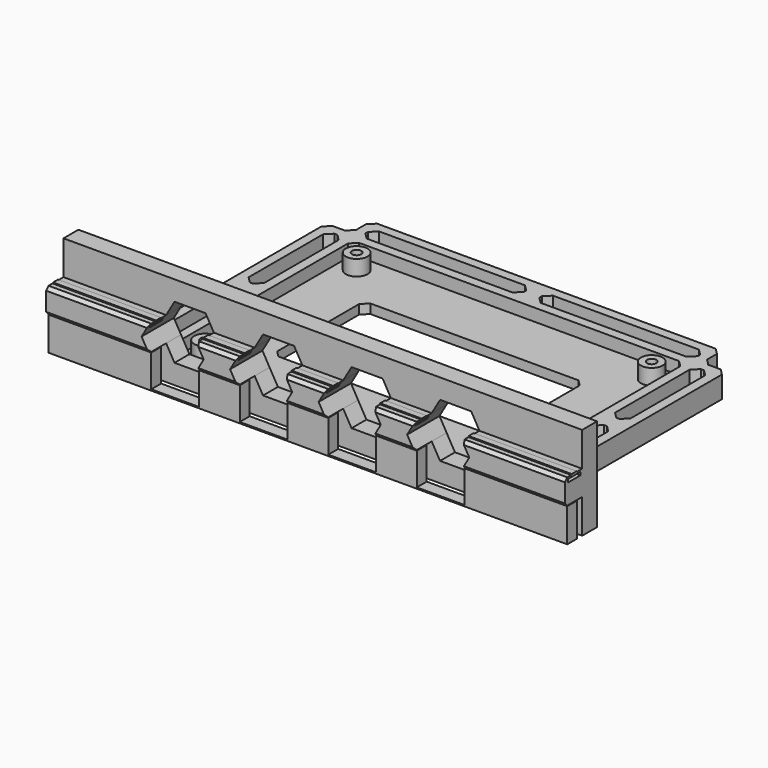
from build123d import *

# Parameters (mm, degrees)
F0_W      = 107
F0_H      = 73
F0_R      = 3.5
F0_W_2    = 71
F0_H_2    = 37
F0_R_2    = 1.5
F0_W_3    = 5
F0_H_3    = 5
F0_W_4    = 3
F0_H_4    = 3
F1_DEPTH  = 3
F2_DEPTH  = 4
F3_DEPTH  = 5
F4_DEPTH  = 27
F6_DEPTH  = 6
F5_W      = 7.5
F5_H      = 8
F5_R      = 3.05
F7_DEPTH  = 7
F8_SIZE   = 1
F9_SIZE   = 2
F11_DEPTH = 167
F12_DEPTH = 7.001
F10_W     = 5
F10_H     = 1
F13_DEPTH = 167.001
F14_W     = 33.0594010768
F14_H     = 4
F14_W_2   = 15.3811978465
F14_W_3   = 13.1188021535
F15_DEPTH = 0.4
F16_DEPTH = 10.8


# Not quite as in the source:
# - an extrude ends at something that could not be found from the text; its depth is read off the source's solid


with BuildPart() as f1:
    # F0 (on Top) → F1 (new body)
    with BuildSketch(Plane.XY):
        Rectangle(F0_W, F0_H)
        with Locations((-47.5, -30.5)):
            Circle(F0_R, mode=Mode.SUBTRACT)
        with Locations((47.5, -30.5)):
            Circle(F0_R, mode=Mode.SUBTRACT)
        Rectangle(F0_W_2, F0_H_2, mode=Mode.SUBTRACT)
        with Locations((-47.5, 30.5)):
            Circle(F0_R, mode=Mode.SUBTRACT)
        with Locations((47.5, 30.5)):
            Circle(F0_R, mode=Mode.SUBTRACT)
        with Locations((-47.5, 30.5)):
            Circle(F0_R)
        with Locations((-47.5, 30.5)):
            Circle(F0_R_2, mode=Mode.SUBTRACT)
        with Locations((-47.5, -30.5)):
            Circle(F0_R)
        with Locations((-47.5, -30.5)):
            Circle(F0_R_2, mode=Mode.SUBTRACT)
        with Locations((47.5, -30.5)):
            Circle(F0_R)
        with Locations((47.5, -30.5)):
            Circle(F0_R_2, mode=Mode.SUBTRACT)
        with Locations((47.5, 30.5)):
            Circle(F0_R)
        with Locations((47.5, 30.5)):
            Circle(F0_R_2, mode=Mode.SUBTRACT)
        Polygon((-53.5, -36.5), (-53.5, 36.5), (-56.5, 36.5), (-56.5, 2.5), (-56.5, -2.5), (-56.5, -36.5), align=None)
        Polygon((-56.5, 36.5), (-56.5, 39.5), (-64.5, 39.5), (-64.5, -36.5), (-61.5, -36.5), (-61.5, -2.5), (-61.5, 2.5), (-61.5, 36.5), align=None)
        with Locations((-59, 0)):
            Rectangle(F0_W_3, F0_H_3)
        with Locations((-55, 38)):
            Rectangle(F0_W_4, F0_H_4)
        Polygon((-53.5, 39.5), (-53.5, 44.5), (-2.5, 44.5), (2.5, 44.5), (53.5, 44.5), (53.5, 39.5), (56.5, 39.5), (56.5, 47.5), (-56.5, 47.5), (-56.5, 39.5), align=None)
        Polygon((-2.5, 39.5), (-53.5, 39.5), (-53.5, 36.5), (53.5, 36.5), (53.5, 39.5), (2.5, 39.5), align=None)
        Polygon((53.5, -36.5), (-53.5, -36.5), (-56.5, -36.5), (-61.5, -36.5), (-64.5, -36.5), (-83.5, -36.5), (-83.5, -42.5), (83.5, -42.5), (83.5, -36.5), (64.5, -36.5), (61.5, -36.5), (56.5, -36.5), align=None)
        with Locations((0, 42)):
            Rectangle(F0_W_3, F0_H_3)
        with Locations((55, 38)):
            Rectangle(F0_W_4, F0_H_4)
        Polygon((56.5, 39.5), (56.5, 36.5), (61.5, 36.5), (61.5, 2.5), (61.5, -2.5), (61.5, -36.5), (64.5, -36.5), (64.5, 39.5), align=None)
        with Locations((59, 0)):
            Rectangle(F0_W_3, F0_H_3)
        Polygon((56.5, 36.5), (53.5, 36.5), (53.5, -36.5), (56.5, -36.5), (56.5, -2.5), (56.5, 2.5), align=None)
    extrude(amount=-F1_DEPTH)

    # F0 (on Top) → F2 (join)
    with BuildSketch(Plane.XY):
        Polygon((-53.5, -36.5), (-53.5, 36.5), (-56.5, 36.5), (-56.5, 2.5), (-56.5, -2.5), (-56.5, -36.5), align=None)
        with Locations((-55, 38)):
            Rectangle(F0_W_4, F0_H_4)
        Polygon((-53.5, 39.5), (-53.5, 44.5), (-2.5, 44.5), (2.5, 44.5), (53.5, 44.5), (53.5, 39.5), (56.5, 39.5), (56.5, 47.5), (-56.5, 47.5), (-56.5, 39.5), align=None)
        Polygon((-56.5, 36.5), (-56.5, 39.5), (-64.5, 39.5), (-64.5, -36.5), (-61.5, -36.5), (-61.5, -2.5), (-61.5, 2.5), (-61.5, 36.5), align=None)
        with Locations((-59, 0)):
            Rectangle(F0_W_3, F0_H_3)
        with Locations((0, 42)):
            Rectangle(F0_W_3, F0_H_3)
        Polygon((-2.5, 39.5), (-53.5, 39.5), (-53.5, 36.5), (53.5, 36.5), (53.5, 39.5), (2.5, 39.5), align=None)
        with Locations((55, 38)):
            Rectangle(F0_W_4, F0_H_4)
        Polygon((56.5, 36.5), (53.5, 36.5), (53.5, -36.5), (56.5, -36.5), (56.5, -2.5), (56.5, 2.5), align=None)
        Polygon((56.5, 39.5), (56.5, 36.5), (61.5, 36.5), (61.5, 2.5), (61.5, -2.5), (61.5, -36.5), (64.5, -36.5), (64.5, 39.5), align=None)
        with Locations((59, 0)):
            Rectangle(F0_W_3, F0_H_3)
    extrude(amount=F2_DEPTH)

    # F0 (on Top) → F3 (join)
    with BuildSketch(Plane.XY):
        with Locations((-47.5, 30.5)):
            Circle(F0_R)
        with Locations((-47.5, 30.5)):
            Circle(F0_R_2, mode=Mode.SUBTRACT)
        with Locations((47.5, 30.5)):
            Circle(F0_R)
        with Locations((47.5, 30.5)):
            Circle(F0_R_2, mode=Mode.SUBTRACT)
        with Locations((47.5, -30.5)):
            Circle(F0_R)
        with Locations((47.5, -30.5)):
            Circle(F0_R_2, mode=Mode.SUBTRACT)
        with Locations((-47.5, -30.5)):
            Circle(F0_R)
        with Locations((-47.5, -30.5)):
            Circle(F0_R_2, mode=Mode.SUBTRACT)
    extrude(amount=F3_DEPTH)

    # F0 (on Top) → F4 (join)
    with BuildSketch(Plane.XY):
        Polygon((53.5, -36.5), (-53.5, -36.5), (-56.5, -36.5), (-61.5, -36.5), (-64.5, -36.5), (-83.5, -36.5), (-83.5, -42.5), (83.5, -42.5), (83.5, -36.5), (64.5, -36.5), (61.5, -36.5), (56.5, -36.5), align=None)
    extrude(amount=F4_DEPTH)

    # F5 (on face) → F6 (cut, through all)
    with BuildSketch(Plane.XZ.offset(42.5)):
        Polygon((-47.75, 20.6602540378), (-50.4405989232, 16), (-35.0594010768, 16), (-37.75, 20.6602540378), align=None)
        Polygon((-35.0594010768, 16), (-50.4405989232, 16), (-52.75, 12), (-50.4405989232, 8), (-35.0594010768, 8), (-32.75, 12), align=None)
        Polygon((-35.0594010768, 8), (-50.4405989232, 8), (-47.75, 3.3397459622), (-37.75, 3.3397459622), align=None)
        Polygon((-6.5594010768, 8), (-21.9405989232, 8), (-19.25, 3.3397459622), (-9.25, 3.3397459622), align=None)
        Polygon((-6.5594010768, 16), (-21.9405989232, 16), (-24.25, 12), (-21.9405989232, 8), (-6.5594010768, 8), (-4.25, 12), align=None)
        Polygon((-19.25, 20.6602540378), (-21.9405989232, 16), (-6.5594010768, 16), (-9.25, 20.6602540378), align=None)
        Polygon((9.25, 20.6602540378), (6.5594010768, 16), (21.9405989232, 16), (19.25, 20.6602540378), align=None)
        Polygon((21.9405989232, 16), (6.5594010768, 16), (4.25, 12), (6.5594010768, 8), (21.9405989232, 8), (24.25, 12), align=None)
        Polygon((21.9405989232, 8), (6.5594010768, 8), (9.25, 3.3397459622), (19.25, 3.3397459622), align=None)
        Polygon((47.75, 3.3397459622), (50.4405989232, 8), (35.0594010768, 8), (37.75, 3.3397459622), align=None)
        Polygon((52.75, 12), (50.4405989232, 16), (35.0594010768, 16), (32.75, 12), (35.0594010768, 8), (50.4405989232, 8), align=None)
        Polygon((35.0594010768, 16), (50.4405989232, 16), (47.75, 20.6602540378), (37.75, 20.6602540378), align=None)
    extrude(amount=-F6_DEPTH, mode=Mode.SUBTRACT)

    # F5 (on face) → F7 (join)
    with BuildSketch(Plane.XZ.offset(42.5)):
        with Locations((-79.75, 12)):
            Rectangle(F5_W, F5_H)
        with Locations((79.75, 12)):
            Rectangle(F5_W, F5_H)
        Polygon((61, 8), (61, 16), (50.4405989232, 16), (52.75, 12), (50.4405989232, 8), align=None)
        Polygon((32.75, 12), (35.0594010768, 16), (21.9405989232, 16), (24.25, 12), (21.9405989232, 8), (35.0594010768, 8), align=None)
        Polygon((6.5594010768, 16), (-6.5594010768, 16), (-4.25, 12), (-6.5594010768, 8), (6.5594010768, 8), (4.25, 12), align=None)
        Polygon((-21.9405989232, 16), (-35.0594010768, 16), (-32.75, 12), (-35.0594010768, 8), (-21.9405989232, 8), (-24.25, 12), align=None)
        Polygon((-50.4405989232, 16), (-61, 16), (-61, 8), (-50.4405989232, 8), (-52.75, 12), align=None)
        with BuildLine():
            ThreePointArc((64.5808164115, 8), (62.9, 12), (64.5808164115, 16))
            Line((64.5808164115, 16), (61, 16))
            Line((61, 16), (61, 8))
            Line((61, 8), (64.5808164115, 8))
        make_face()
        with BuildLine():
            ThreePointArc((74.1, 12), (73.6627235107, 14.1693976013), (72.4191835885, 16))
            Line((72.4191835885, 16), (64.5808164115, 16))
            ThreePointArc((64.5808164115, 16), (62.9, 12), (64.5808164115, 8))
            Line((64.5808164115, 8), (72.4191835885, 8))
            ThreePointArc((72.4191835885, 8), (73.6627235107, 9.8306023987), (74.1, 12))
        make_face()
        with Locations((68.5, 12)):
            Circle(F5_R, mode=Mode.SUBTRACT)
        with Locations((68.5, 12)):
            Circle(F5_R)
        with BuildLine():
            Line((76, 8), (76, 16))
            Line((76, 16), (72.4191835885, 16))
            ThreePointArc((72.4191835885, 16), (73.6627235107, 14.1693976013), (74.1, 12))
            ThreePointArc((74.1, 12), (73.6627235107, 9.8306023987), (72.4191835885, 8))
            Line((72.4191835885, 8), (76, 8))
        make_face()
        with BuildLine():
            Line((-61, 16), (-64.5808164115, 16))
            ThreePointArc((-64.5808164115, 16), (-63.3372764893, 14.1693976013), (-62.9, 12))
            ThreePointArc((-62.9, 12), (-63.3372764893, 9.8306023987), (-64.5808164115, 8))
            Line((-64.5808164115, 8), (-61, 8))
            Line((-61, 8), (-61, 16))
        make_face()
        with BuildLine():
            Line((-64.5808164115, 16), (-72.4191835885, 16))
            ThreePointArc((-72.4191835885, 16), (-74.1, 12), (-72.4191835885, 8))
            Line((-72.4191835885, 8), (-64.5808164115, 8))
            ThreePointArc((-64.5808164115, 8), (-63.3372764893, 9.8306023987), (-62.9, 12))
            ThreePointArc((-62.9, 12), (-63.3372764893, 14.1693976013), (-64.5808164115, 16))
        make_face()
        with Locations((-68.5, 12)):
            Circle(F5_R, mode=Mode.SUBTRACT)
        with Locations((-68.5, 12)):
            Circle(F5_R)
        with BuildLine():
            Line((-72.4191835885, 16), (-76, 16))
            Line((-76, 16), (-76, 8))
            Line((-76, 8), (-72.4191835885, 8))
            ThreePointArc((-72.4191835885, 8), (-74.1, 12), (-72.4191835885, 16))
        make_face()
    extrude(amount=F7_DEPTH)

    # F8
    f8_edges = [f1.edges().sort_by_distance(p)[0] for p in [
        (-66.970299, -49.5, 8),
        (-66.970299, -49.5, 16),
        (-28.5, -49.5, 16),
        (-28.5, -49.5, 8),
        (0, -49.5, 8),
        (0, -49.5, 16),
        (28.5, -49.5, 16),
        (28.5, -49.5, 8),
        (66.970299, -49.5, 8),
        (66.970299, -49.5, 16),
    ]]
    chamfer(f8_edges, length=F8_SIZE)

    # F9
    f9_edges = [f1.edges().sort_by_distance(p)[0] for p in [
        (35.5, 18.5, -1.5),
        (35.5, -18.5, -1.5),
        (-35.5, 18.5, -1.5),
        (-35.5, -18.5, -1.5),
        (53.5, -36.5, 2),
        (61.5, -36.5, 0.5),
        (53.5, 36.5, 2),
        (61.5, 36.5, 0.5),
        (53.5, 44.5, 0.5),
        (56.5, 36.5, 0.5),
        (2.5, 44.5, 0.5),
        (56.5, -2.5, 0.5),
        (56.5, -36.5, 0.5),
        (56.5, 2.5, 0.5),
        (61.5, 2.5, 0.5),
        (53.5, 39.5, 0.5),
        (2.5, 39.5, 0.5),
        (-2.5, 44.5, 0.5),
        (-56.5, 36.5, 0.5),
        (-56.5, -2.5, 0.5),
        (-61.5, -2.5, 0.5),
        (-61.5, 36.5, 0.5),
        (-53.5, 44.5, 0.5),
        (-53.5, 39.5, 0.5),
        (-61.5, -36.5, 0.5),
        (-61.5, 2.5, 0.5),
        (-56.5, 2.5, 0.5),
        (-56.5, -36.5, 0.5),
        (-2.5, 39.5, 0.5),
        (-53.5, 36.5, 2),
        (-53.5, -36.5, 2),
        (64.5, 39.5, 0.5),
        (56.5, 47.5, 0.5),
        (56.5, 39.5, 0.5),
        (64.5, -36.5, 0.5),
        (-56.5, 47.5, 0.5),
        (-56.5, 39.5, 0.5),
        (-64.5, 39.5, 0.5),
        (-64.5, -36.5, 0.5),
        (61.5, -2.5, 0.5),
    ]]
    chamfer(f9_edges, length=F9_SIZE)

    # F10 (on face) → F11 (join, through all)
    with BuildSketch(Plane(origin=(-83.5, 0, 0), x_dir=(0, -1, 0), z_dir=(-1, 0, 0))):
        Polygon((44.7, 16.2), (44.5, 16), (46.9, 16), (46.7, 16.2), align=None)
    extrude(amount=-F11_DEPTH)

    # F5 (on face) → F12 (cut, through all)
    with BuildSketch(Plane.XZ.offset(42.5)):
        Polygon((-47.75, 20.6602540378), (-50.4405989232, 16), (-35.0594010768, 16), (-37.75, 20.6602540378), align=None)
        Polygon((-19.25, 20.6602540378), (-21.9405989232, 16), (-6.5594010768, 16), (-9.25, 20.6602540378), align=None)
        Polygon((9.25, 20.6602540378), (6.5594010768, 16), (21.9405989232, 16), (19.25, 20.6602540378), align=None)
        Polygon((35.0594010768, 16), (50.4405989232, 16), (47.75, 20.6602540378), (37.75, 20.6602540378), align=None)
    extrude(amount=F12_DEPTH, mode=Mode.SUBTRACT)

    # F10 (on face) → F13 (cut, through all)
    with BuildSketch(Plane(origin=(-83.5, 0, 0), x_dir=(0, -1, 0), z_dir=(-1, 0, 0))):
        with Locations((45.7, 14.9)):
            Rectangle(F10_W, F10_H)
    extrude(amount=-F13_DEPTH, mode=Mode.SUBTRACT)


with BuildPart() as f15:
    # F14 (on face) → F15 (new body)
    with BuildSketch(Plane(origin=(0, 0, -3), x_dir=(1, 0, 0), z_dir=(0, 0, -1))):
        with Locations((-66.9702994616, 46.5)):
            Rectangle(F14_W, F14_H)
        with Locations((-42.75, 46.5)):
            Rectangle(F14_W_2, F14_H)
        with Locations((-28.5, 46.5)):
            Rectangle(F14_W_3, F14_H)
        with Locations((-14.25, 46.5)):
            Rectangle(F14_W_2, F14_H)
        with Locations((0, 46.5)):
            Rectangle(F14_W_3, F14_H)
        with Locations((14.25, 46.5)):
            Rectangle(F14_W_2, F14_H)
        with Locations((28.5, 46.5)):
            Rectangle(F14_W_3, F14_H)
        with Locations((42.75, 46.5)):
            Rectangle(F14_W_2, F14_H)
        with Locations((66.9702994616, 46.5)):
            Rectangle(F14_W, F14_H)
    extrude(amount=-F15_DEPTH)

    # F14 (on face) → F16 (join, through all)
    with BuildSketch(Plane(origin=(0, 0, -3), x_dir=(1, 0, 0), z_dir=(0, 0, -1))):
        with Locations((-66.9702994616, 46.5)):
            Rectangle(F14_W, F14_H)
        with Locations((66.9702994616, 46.5)):
            Rectangle(F14_W, F14_H)
        with Locations((-28.5, 46.5)):
            Rectangle(F14_W_3, F14_H)
        with Locations((0, 46.5)):
            Rectangle(F14_W_3, F14_H)
        with Locations((28.5, 46.5)):
            Rectangle(F14_W_3, F14_H)
    extrude(amount=-F16_DEPTH)


solid = Compound([f1.part, f15.part])
